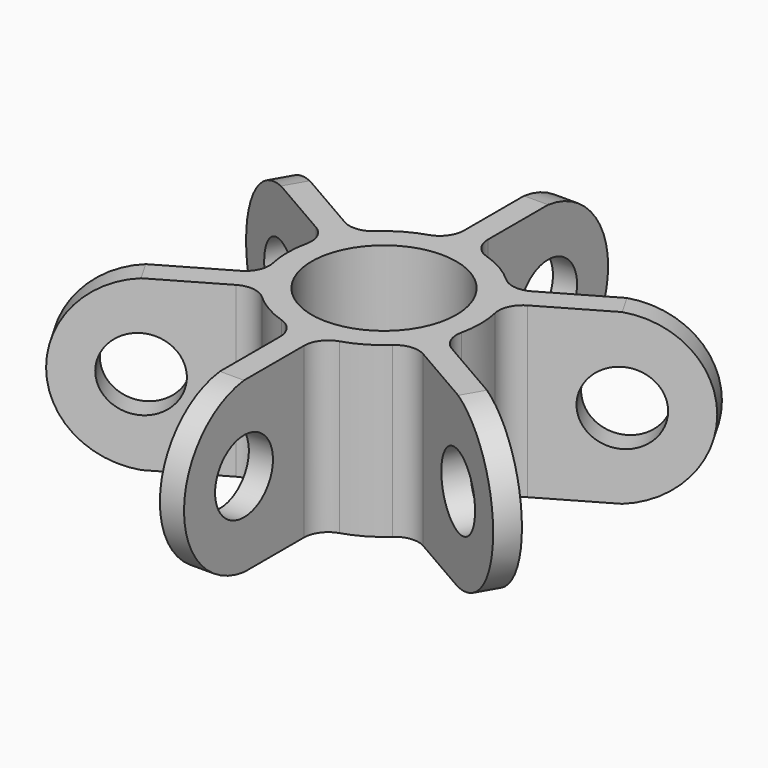
from build123d import *

# Parameters (mm, degrees)
F0_R            = 4.7625
F1_DEPTH        = 11.1125
F2_R            = 1.5875
F3_R            = 2.38125
F4_DEPTH        = 23.6698249306
F4_COPIES_COUNT = 6


# Not quite as in the source:
# - a pattern or mirror of a feature is missing from the dataset's text; its kind, count and spacing are read off the source's solid


with BuildPart() as f1:
    # F0 (on Top) → F1 (new body)
    with BuildSketch(Plane.XY):
        with BuildLine():
            Line((-0.79375, 17.4444508996), (-0.79375, 6.3001953095))
            ThreePointArc((-0.79375, 6.3001953095), (-3.175, 5.499261314), (-5.0592541868, 3.837505319))
            Line((-5.0592541868, 3.837505319), (-14.7104626341, 9.409633114))
            ThreePointArc((-14.7104626341, 9.409633114), (-15.1229686136, 8.73125), (-15.5042126341, 8.0348177855))
            Line((-15.5042126341, 8.0348177855), (-5.8530041868, 2.4626899905))
            ThreePointArc((-5.8530041868, 2.4626899905), (-6.35, 0), (-5.8530041868, -2.4626899905))
            Line((-5.8530041868, -2.4626899905), (-15.5042126341, -8.0348177855))
            ThreePointArc((-15.5042126341, -8.0348177855), (-15.1229686136, -8.73125), (-14.7104626341, -9.409633114))
            Line((-14.7104626341, -9.409633114), (-5.0592541868, -3.837505319))
            ThreePointArc((-5.0592541868, -3.837505319), (-3.175, -5.499261314), (-0.79375, -6.3001953095))
            Line((-0.79375, -6.3001953095), (-0.79375, -17.4444508996))
            ThreePointArc((-0.79375, -17.4444508996), (0, -17.4625), (0.79375, -17.4444508996))
            Line((0.79375, -17.4444508996), (0.79375, -6.3001953095))
            ThreePointArc((0.79375, -6.3001953095), (3.175, -5.499261314), (5.0592541868, -3.837505319))
            Line((5.0592541868, -3.837505319), (14.7104626341, -9.409633114))
            ThreePointArc((14.7104626341, -9.409633114), (15.1229686136, -8.73125), (15.5042126341, -8.0348177855))
            Line((15.5042126341, -8.0348177855), (5.8530041868, -2.4626899905))
            ThreePointArc((5.8530041868, -2.4626899905), (6.35, 0), (5.8530041868, 2.4626899905))
            Line((5.8530041868, 2.4626899905), (15.5042126341, 8.0348177855))
            ThreePointArc((15.5042126341, 8.0348177855), (15.1229686136, 8.73125), (14.7104626341, 9.409633114))
            Line((14.7104626341, 9.409633114), (5.0592541868, 3.837505319))
            ThreePointArc((5.0592541868, 3.837505319), (3.175, 5.499261314), (0.79375, 6.3001953095))
            Line((0.79375, 6.3001953095), (0.79375, 17.4444508996))
            ThreePointArc((0.79375, 17.4444508996), (0, 17.4625), (-0.79375, 17.4444508996))
        make_face()
        Circle(F0_R, mode=Mode.SUBTRACT)
    extrude(amount=F1_DEPTH)

    # F2
    f2_edges = [f1.edges().sort_by_distance(p)[0] for p in [
        (-5.059254, 3.837505, 5.55625),
        (0.79375, 6.300195, 5.55625),
        (5.059254, 3.837505, 5.55625),
        (5.853004, -2.46269, 5.55625),
        (5.853004, 2.46269, 5.55625),
        (0.79375, -6.300195, 5.55625),
        (5.059254, -3.837505, 5.55625),
        (-0.79375, -6.300195, 5.55625),
        (-5.059254, -3.837505, 5.55625),
        (-5.853004, -2.46269, 5.55625),
        (-5.853004, 2.46269, 5.55625),
        (-0.79375, 6.300195, 5.55625),
    ]]
    fillet(f2_edges, radius=F2_R)

    # F3 (on face) → F4 (cut, through all)
    with BuildSketch(Plane(origin=(0.396875, -0.6874076643, 0), x_dir=(0.8660254038, 0.5, 0), z_dir=(0.5, -0.8660254038, 0))):
        with Locations((12.5081716554, 5.55625)):
            Circle(F3_R)
        with BuildLine():
            ThreePointArc((12.5081716554, 11.1125), (17.4444508996, 5.55625), (12.5081716554, 0))
            Line((12.5081716554, 0), (12.5081716554, -1.8244276289))
            Line((12.5081716554, -1.8244276289), (18.7674891204, -1.8244276289))
            Line((18.7674891204, -1.8244276289), (18.7674891204, 12.5710107386))
            Line((18.7674891204, 12.5710107386), (12.5081716554, 12.5710107386))
            Line((12.5081716554, 12.5710107386), (12.5081716554, 11.1125))
        make_face()
    f4 = extrude(amount=-F4_DEPTH, mode=Mode.SUBTRACT)

    # F4_copies: F4 ×6 about axis
    f4_copies_axis = Axis((0, 0, 0), (0, 0, 1))
    for i in range(1, F4_COPIES_COUNT):
        add(f4.rotate(f4_copies_axis, i * 360 / F4_COPIES_COUNT), mode=Mode.SUBTRACT)


solid = f1.part
